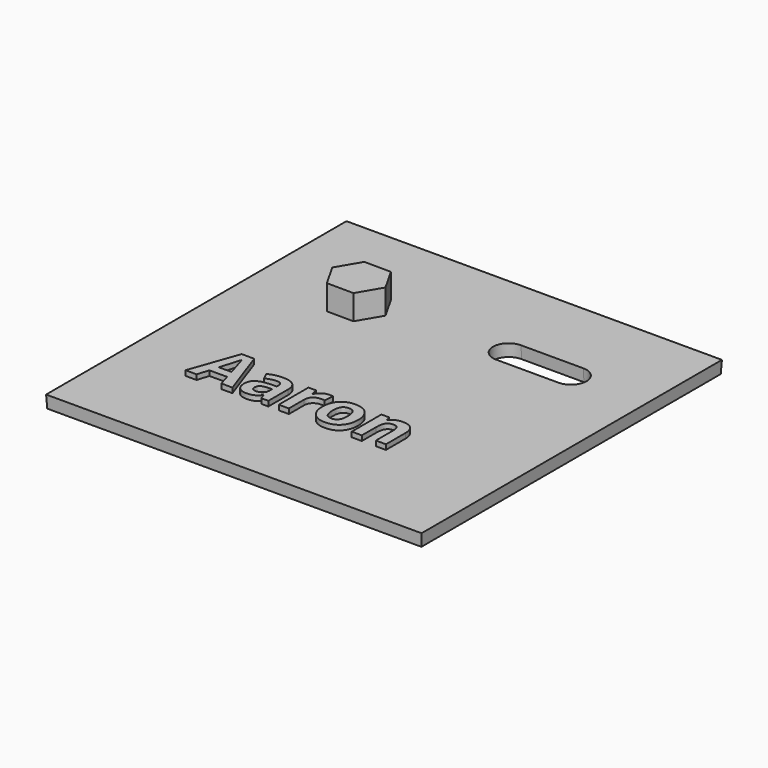
from build123d import *

# Parameters (mm, degrees)
F0_W         = 75
F0_H         = 75
F1_DEPTH     = 5
F1_TAPER     = -3
F2_TEXT_SIZE = 27.2403471172
F3_DEPTH     = 2
F5_DEPTH     = 9.9485572428


# Not quite as in the source:
# - Text() gives the source's letters only with a copy of the font that has no kerning and outlines rounded to 1/6400 em; it was checked with that copy


with BuildPart() as f1:
    # F0 (on Top) → F1 (new body)
    with BuildSketch(Plane.XY):
        with Locations((-37.5, -37.5)):
            Rectangle(F0_W, F0_H)
        with Locations((37.5, -37.5)):
            Rectangle(F0_W, F0_H)
        with Locations((-37.5, 37.5)):
            Rectangle(F0_W, F0_H)
        with Locations((37.5, 37.5)):
            Rectangle(F0_W, F0_H)
        with BuildLine():
            Line((44.9799537659, 30.9560877681), (19.9799537659, 30.9560877681))
            ThreePointArc((19.9799537659, 30.9560877681), (13.4799537659, 37.4560877681), (19.9799537659, 43.9560877681))
            Line((19.9799537659, 43.9560877681), (44.9799537659, 43.9560877681))
            ThreePointArc((44.9799537659, 43.9560877681), (51.4799537659, 37.4560877681), (44.9799537659, 30.9560877681))
        make_face(mode=Mode.SUBTRACT)
    extrude(amount=F1_DEPTH, taper=F1_TAPER)

    # F2 (on face) → F3 (join)
    with BuildSketch(Plane.XY.offset(5)):
        with Locations((-49.0589886904, -38.1327420473)):
            Text('Aaron', F2_TEXT_SIZE, font='Open Sans', font_style=FontStyle.BOLD, text_align=(TextAlign.LEFT, TextAlign.BOTTOM))
    extrude(amount=F3_DEPTH)

    # F4 (on face) → F5 (join)
    with BuildSketch(Plane.XY.offset(5)):
        Polygon((-31.1373804135, 23.612273293), (-25.69931373, 32.8606031835), (-30.989569016, 42.1942720242), (-41.7178909855, 42.2796109743), (-47.155957669, 33.0312810838), (-41.865702383, 23.6976122432), align=None)
    extrude(amount=F5_DEPTH)


solid = f1.part
